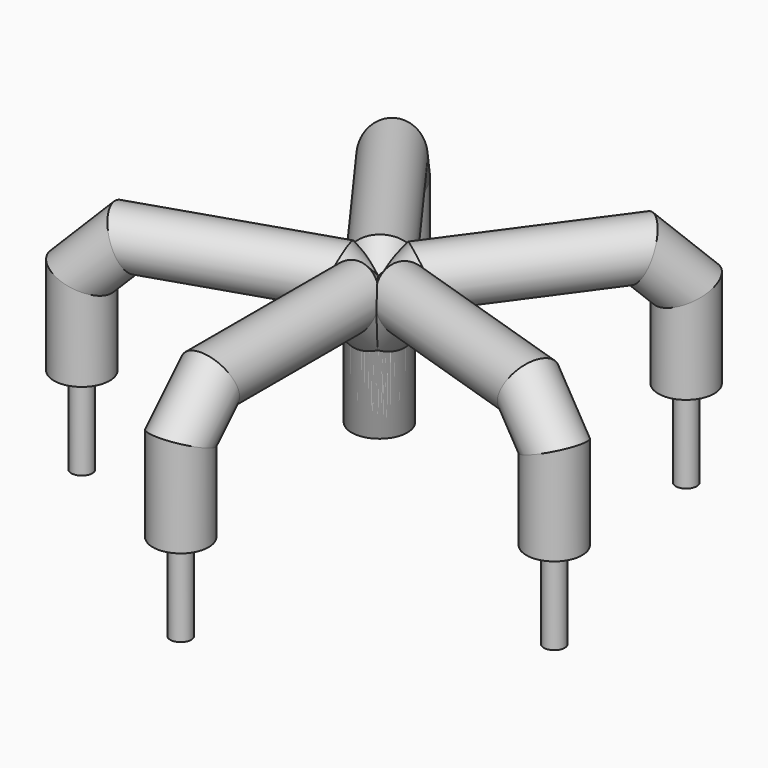
from build123d import *

# Parameters (mm, degrees)
F0_R     = 8
F4_R     = 2.9999983311
F5_DEPTH = 25
F6_COUNT = 5


with BuildPart() as f2:
    # F2: sweep along a path in F1
    with BuildLine(Plane.YZ) as f2_path:
        Line((0, 70), (25, 70))
        Line((25, 70), (35.6066017178, 59.3933982822))
        Line((35.6066017178, 59.3933982822), (35.6066017178, 34.3933982822))
    # F0 (on Front) → F2 (sweep)
    with BuildSketch(Plane.XZ):
        with Locations((70, 70)):
            Circle(F0_R)
    sweep(path=f2_path.line, transition=Transition.RIGHT)

    # F3: F2 across plane


with BuildPart() as f2_1:
    add(f2.part)
    add(f2.part.mirror(Plane.XZ))

    # F4 (on face) → F5 (join)
    with BuildSketch(Plane(origin=(0, 0, 34.3933982822), x_dir=(1, 0, 0), z_dir=(0, 0, -1))):
        with Locations((70, 35.6066017178)):
            Circle(F4_R)
    extrude(amount=F5_DEPTH)


with BuildPart() as f6_1:
    # F6: instance of F2
    add(f2_1.part.rotate(Axis((70, 35.6066017178, 59.3933982822), (0, 0, -1)), 1 * 360 / F6_COUNT))


with BuildPart() as f6_2:
    # F6: instance of F2
    add(f2_1.part.rotate(Axis((70, 35.6066017178, 59.3933982822), (0, 0, -1)), 2 * 360 / F6_COUNT))


with BuildPart() as f6_3:
    # F6: instance of F2
    add(f2_1.part.rotate(Axis((70, 35.6066017178, 59.3933982822), (0, 0, -1)), 3 * 360 / F6_COUNT))


with BuildPart() as f6_4:
    # F6: instance of F2
    add(f2_1.part.rotate(Axis((70, 35.6066017178, 59.3933982822), (0, 0, -1)), 4 * 360 / F6_COUNT))


solid = Compound([f2_1.part, f6_1.part, f6_2.part, f6_3.part, f6_4.part])
